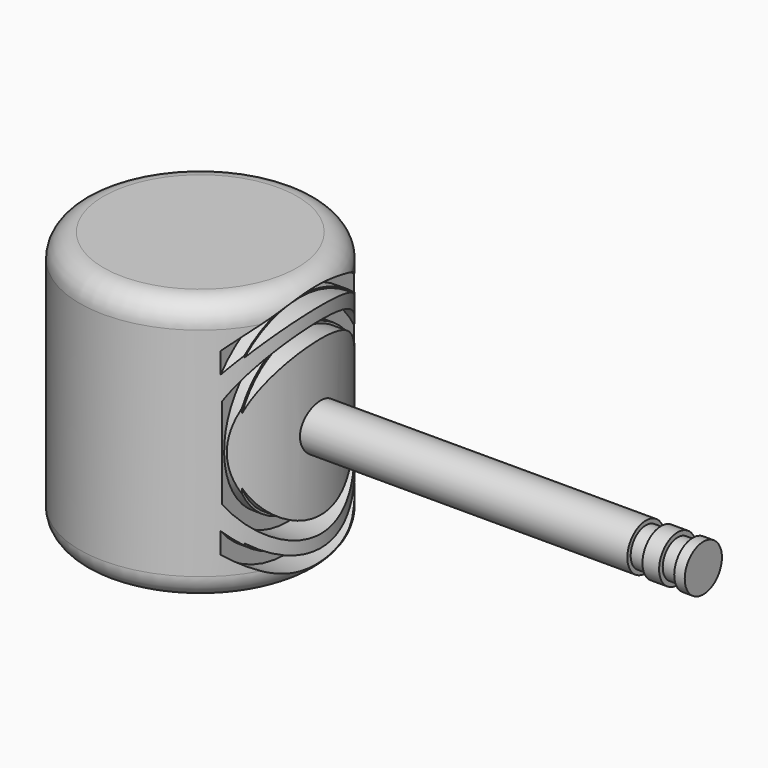
from build123d import *

# Parameters (mm, degrees)
F0_W   = 25.4
F0_H   = 55.7187045847
F2_W   = 118.6923170462
F2_H   = 4.8982012086
F4_W   = 3.185287118
F4_H   = 12.2274383903
F4_W_2 = 20.8224356174
F4_H_2 = 3.0317753553


# Not quite as in the source:
# - a fillet or chamfer that OpenCascade refuses, or shapes differently, is made with other operations: its cross-section is extruded or revolved along the edge and cut away or added


with BuildPart() as f1:
    # F0 (on Front) → F1 (revolve)
    with BuildSketch(Plane.XZ):
        Rectangle(F0_W, F0_H)
    revolve(axis=Axis((12.7, 0, 0), (0, 0, -1)))

    # F2 (on Front) → F3 (revolve)
    with BuildSketch(Plane.XZ):
        with Locations((59.3461585231, -2.4491006043)):
            Rectangle(F2_W, F2_H)
    revolve(axis=Axis((59.3461585231, 0, 0), (-1, 0, 0)))

    # F4 (on Front) → F6 (revolve, cut)
    with BuildSketch(Plane.XZ):
        with Locations((114.8856207728, -10.0567732006)):
            Rectangle(F4_W, F4_H)
        with Locations((108.191460371, -10.1317744702)):
            Rectangle(F4_W, F4_H)
        with Locations((43.9788103104, -24.0039676428)):
            Rectangle(F4_W_2, F4_H_2)
        with Locations((43.7408648431, -17.8672224283)):
            Rectangle(F4_W_2, F4_H_2)
        with Locations((41.584610939, 18.3283146471)):
            Rectangle(F4_W_2, F4_H_2)
        with Locations((41.4398871362, 24.3011359125)):
            Rectangle(F4_W_2, F4_H_2)
    revolve(axis=Axis((52.5897778571, 0, 0), (1, 0, 0)), mode=Mode.SUBTRACT)

    # F7: fillet of radius 5 on 1 edges, made by hand

    # F7_s1 → F7_t2 (revolve, cut)
    with BuildSketch(Plane.XZ):
        with BuildLine():
            ThreePointArc((-12.7, -22.8593522923), (-11.2355339059, -26.3948861983), (-7.7, -27.8593522923))
            Line((-7.7, -27.8593522923), (-12.7, -27.8593522923))
            Line((-12.7, -27.8593522923), (-12.7, -22.8593522923))
        make_face()
    revolve(axis=Axis((12.7, 0, -27.8593522923), (0, 0, -1)), mode=Mode.SUBTRACT)

    # F8: fillet of radius 5 on 1 edges, made by hand

    # F8_s1 → F8_t2 (revolve, cut)
    with BuildSketch(Plane.XZ):
        with BuildLine():
            ThreePointArc((-7.7, 27.8593522923), (-11.2355339059, 26.3948861983), (-12.7, 22.8593522923))
            Line((-12.7, 22.8593522923), (-12.7, 27.8593522923))
            Line((-12.7, 27.8593522923), (-7.7, 27.8593522923))
        make_face()
    revolve(axis=Axis((12.7, 0, 27.8593522923), (0, 0, -1)), mode=Mode.SUBTRACT)


solid = f1.part
